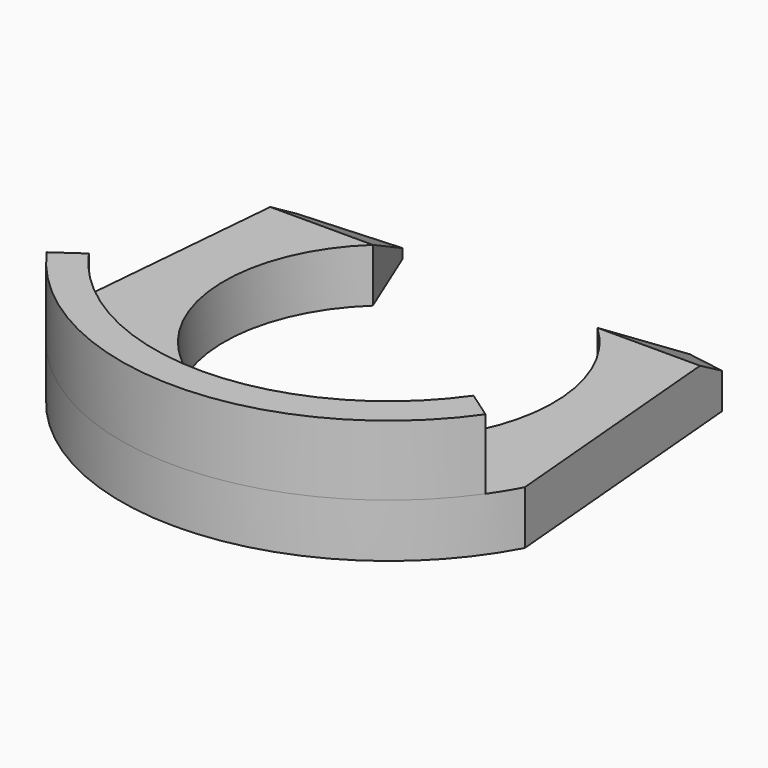
from build123d import *

# Parameters (mm, degrees)
F2_DEPTH = 1.3
F4_DEPTH = 1.7
F6_DEPTH = 12.5


# Not quite as in the source:
# - a feature of the source that left no trace in its solid (it failed there, or was rolled back) is left out


with BuildPart() as f2:
    # F1 (on Top) → F2 (new body)
    with BuildSketch(Plane.XY):
        with BuildLine():
            Line((-5.1537473182, 3.6727124144), (-5.7416372565, -3.0469003289))
            ThreePointArc((-5.7416372565, -3.0469003289), (0, -6.5), (5.7416372565, -3.0469003289))
            Line((5.7416372565, -3.0469003289), (5.1537473182, 3.6727124144))
            Line((5.1537473182, 3.6727124144), (3.4859795486, 4.7765922388))
            Line((3.4859795486, 4.7765922388), (2.7272692442, 2.9260899627))
            ThreePointArc((2.7272692442, 2.9260899627), (0, -4), (-2.7272692442, 2.9260899627))
            Line((-2.7272692442, 2.9260899627), (-3.4859795486, 4.7765922388))
            Line((-3.4859795486, 4.7765922388), (-5.1537473182, 3.6727124144))
        make_face()
    extrude(amount=F2_DEPTH)

    # F3 (on face) → F4 (join)
    with BuildSketch(Plane.XY.offset(1.3)):
        with BuildLine():
            Line((-4.6721311475, -3.2651478589), (-5.3278688525, -3.723414225))
            ThreePointArc((-5.3278688525, -3.723414225), (0, -6.5), (5.3278688525, -3.723414225))
            Line((5.3278688525, -3.723414225), (4.6721311475, -3.2651478589))
            ThreePointArc((4.6721311475, -3.2651478589), (0, -5.7), (-4.6721311475, -3.2651478589))
        make_face()
    extrude(amount=F4_DEPTH)

    # F5 (on Right) → F6 (cut, symmetric)
    with BuildSketch(Plane.YZ):
        Polygon((6.7765922388, 1.3), (2.9260899627, 1.3), (6.7765922388, -0.9230885256), align=None)
    extrude(amount=F6_DEPTH, both=True, mode=Mode.SUBTRACT)


solid = f2.part
